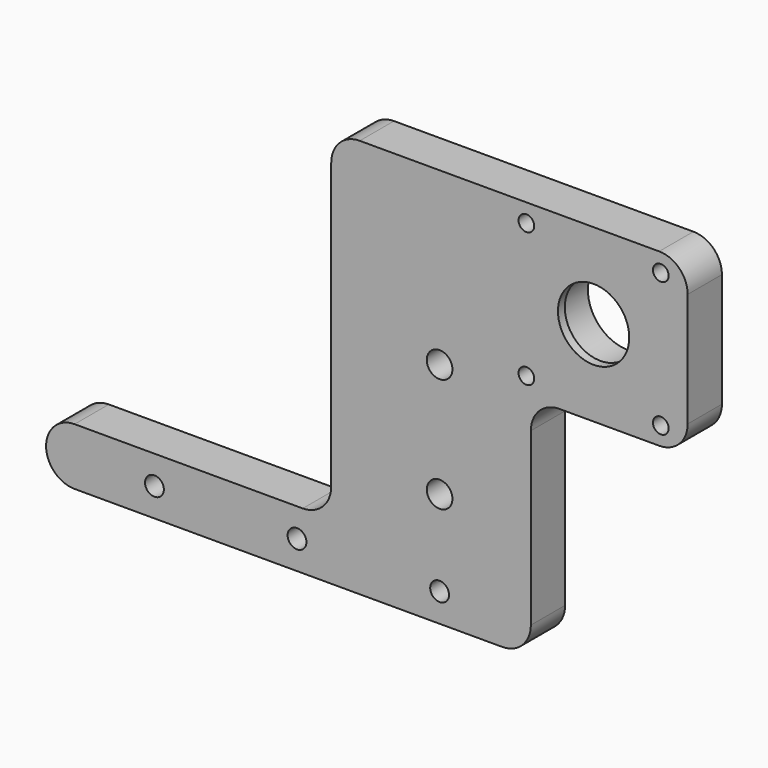
from build123d import *

# Parameters (mm, degrees)
F1_DEPTH       = 15
F2_D           = 9
F3_D           = 6.6
F4_R           = 9.99999
F5_D           = 28
F6_D           = 5.5
F6_CBORE_D     = 9.75
F6_CBORE_DEPTH = 5
F7_W           = 40
F7_H           = 80
F8_DEPTH       = 5
F11_R          = 14
F11_R_2        = 12.5
F12_DEPTH      = 3


# Not quite as in the source:
# - a fillet or chamfer is up to 0.001 mm smaller than in the source, because OpenCascade refuses the exact size


with BuildPart() as f1:
    # F0 (on Front) → F1 (new body)
    with BuildSketch(Plane.XZ):
        Polygon((62.0740194619, 20.9148037434), (-57.9259805381, 20.9148037434), (-62.9259805381, 20.9148037434), (-62.9259805381, -39.0851962566), (-57.9259805381, -39.0851962566), (-7.9259805381, -39.0851962566), (-7.9259805381, -119.0851962566), (162.0740194619, -119.0851962566), (162.0740194619, -99.0851962566), (62.0740194619, -99.0851962566), align=None)
    extrude(amount=F1_DEPTH)

    # F2 (through all)
    with Locations(Plane(origin=(0, 0, 0), x_dir=(1, 0, 0), z_dir=(0, 1, 0))):
        with Locations((24.0740194619, 79.0851962566), (24.0740194619, 39.0851962566)):
            Hole(F2_D / 2)

    # F3 (through all)
    with Locations(Plane(origin=(0, 0, 0), x_dir=(1, 0, 0), z_dir=(0, 1, 0))):
        with Locations((24.0740194619, 109.0851962566), (74.0740194619, 109.0851962566), (124.0740194619, 109.0851962566)):
            Hole(F3_D / 2)

    # F4 (radius 10 in the source; OpenCascade refuses exactly that, so slightly less here)
    f4_edges = [f1.edges().sort_by_distance(p)[0] for p in [
        (62.074019, -7.5, 20.914804),
        (62.074019, -7.5, -99.085196),
        (162.074019, -7.5, -119.085196),
        (162.074019, -7.5, -99.085196),
        (-7.925981, -7.5, -119.085196),
        (-7.925981, -7.5, -39.085196),
        (-62.925981, -7.5, 20.914804),
        (-62.925981, -7.5, -39.085196),
    ]]
    fillet(f4_edges, radius=F4_R)

    # F5 (through all)
    with Locations(Plane(origin=(0, 0, 0), x_dir=(1, 0, 0), z_dir=(0, 1, 0))):
        with Locations((-29.9259805381, 9.0851962566)):
            Hole(F5_D / 2)

    # F6 (through all)
    with Locations(Plane(origin=(0, 0, 0), x_dir=(1, 0, 0), z_dir=(0, 1, 0))):
        with Locations((-53.4959805381, -14.4848037434), (-6.3559805381, -14.4848037434), (-6.3559805381, 32.6551962566), (-53.4959805381, 32.6551962566)):
            CounterBoreHole(F6_D / 2, F6_CBORE_D / 2, F6_CBORE_DEPTH)

    # F7 (on face) → F8 (cut)
    with BuildSketch(Plane.XZ):
        with Locations((24.0740194619, -59.0851962566)):
            Rectangle(F7_W, F7_H)
    extrude(amount=F8_DEPTH, mode=Mode.SUBTRACT)


with BuildPart() as f10_1:
    # F10: instance of F1
    add(f1.part.mirror(Plane.YZ.offset(-100)))

    # F11 (on face) → F12 (join)
    with BuildSketch(Plane.XZ.offset(15)):
        with Locations((-170.0740194619, -9.0851962566)):
            Circle(F11_R)
        with Locations((-170.0740194619, -9.0851962566)):
            Circle(F11_R_2, mode=Mode.SUBTRACT)
    extrude(amount=-F12_DEPTH)


solid = f10_1.part
